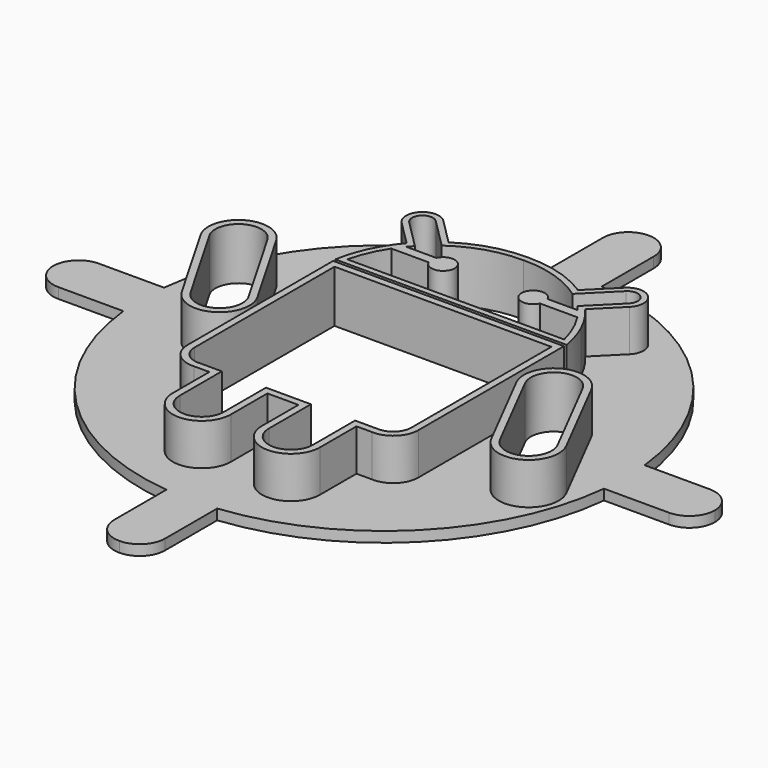
from build123d import *

# Parameters (mm, degrees)
F1_DEPTH = 3
F3_DEPTH = 25
F6_DEPTH = 12
F7_DEPTH = 12
F8_SCALE = 0.5


# Not quite as in the source:
# - a feature of the source that left no trace in its solid (it failed there, or was rolled back) is left out
# - a feature names something its author has since deleted; it is built from what else it names


with BuildPart() as f1:
    # F0 (on Top) → F1 (new body)
    with BuildSketch(Plane.XY):
        with BuildLine():
            ThreePointArc((69.1465082783, -7.3148026297), (69.4358131239, -3.6624855503), (69.532337402, 0))
            ThreePointArc((69.532337402, 0), (69.4358131239, 3.6624855503), (69.1465082783, 7.3148026297))
            ThreePointArc((69.1465082783, 7.3148026297), (49.1667872887, 49.1667872887), (7.3148026297, 69.1465082783))
            ThreePointArc((7.3148026297, 69.1465082783), (0, 69.532337402), (-7.3148026297, 69.1465082783))
            ThreePointArc((-7.3148026297, 69.1465082783), (-49.1667872887, 49.1667872887), (-69.1465082783, 7.3148026297))
            ThreePointArc((-69.1465082783, 7.3148026297), (-69.532337402, 0), (-69.1465082783, -7.3148026297))
            ThreePointArc((-69.1465082783, -7.3148026297), (-49.1667872887, -49.1667872887), (-7.3148026297, -69.1465082783))
            ThreePointArc((-7.3148026297, -69.1465082783), (0, -69.532337402), (7.3148026297, -69.1465082783))
            ThreePointArc((7.3148026297, -69.1465082783), (49.1667872887, -49.1667872887), (69.1465082783, -7.3148026297))
        make_face()
        with BuildLine():
            ThreePointArc((69.1465082783, 7.3148026297), (69.4358131239, 3.6624855503), (69.532337402, 0))
            ThreePointArc((69.532337402, 0), (69.4358131239, -3.6624855503), (69.1465082783, -7.3148026297))
            Line((69.1465082783, -7.3148026297), (87.8831749798, -7.3148026297))
            ThreePointArc((87.8831749798, -7.3148026297), (93.0555215223, -5.1723465425), (95.1979776095, 0))
            ThreePointArc((95.1979776095, 0), (93.0555215223, 5.1723465425), (87.8831749798, 7.3148026297))
            Line((87.8831749798, 7.3148026297), (69.1465082783, 7.3148026297))
        make_face()
        with BuildLine():
            ThreePointArc((-7.3148026297, 69.1465082783), (0, 69.532337402), (7.3148026297, 69.1465082783))
            Line((7.3148026297, 69.1465082783), (7.3148026297, 87.8831749798))
            ThreePointArc((7.3148026297, 87.8831749798), (5.1723465425, 93.0555215223), (0, 95.1979776095))
            ThreePointArc((0, 95.1979776095), (-5.1723465425, 93.0555215223), (-7.3148026297, 87.8831749798))
            Line((-7.3148026297, 87.8831749798), (-7.3148026297, 69.1465082783))
        make_face()
        with BuildLine():
            Line((7.3148026297, -87.8831749798), (7.3148026297, -69.1465082783))
            ThreePointArc((7.3148026297, -69.1465082783), (0, -69.532337402), (-7.3148026297, -69.1465082783))
            Line((-7.3148026297, -69.1465082783), (-7.3148026297, -87.8831749798))
            ThreePointArc((-7.3148026297, -87.8831749798), (-5.1723465425, -93.0555215223), (0, -95.1979776095))
            ThreePointArc((0, -95.1979776095), (5.1723465425, -93.0555215223), (7.3148026297, -87.8831749798))
        make_face()
        with BuildLine():
            ThreePointArc((-69.1465082783, -7.3148026297), (-69.532337402, 0), (-69.1465082783, 7.3148026297))
            Line((-69.1465082783, 7.3148026297), (-87.8831749798, 7.3148026297))
            ThreePointArc((-87.8831749798, 7.3148026297), (-93.0555215223, 5.1723465425), (-95.1979776095, 0))
            ThreePointArc((-95.1979776095, 0), (-93.0555215223, -5.1723465425), (-87.8831749798, -7.3148026297))
            Line((-87.8831749798, -7.3148026297), (-69.1465082783, -7.3148026297))
        make_face()
    extrude(amount=F1_DEPTH)

    # F2 (on face) → F3 (cut)
    with BuildSketch(Plane.XY.offset(3)):
        with BuildLine():
            ThreePointArc((-51.2002213642, 22.0671218808), (-60.2199302878, 24.4839456028), (-62.6367540099, 15.4642366792))
            Line((-62.6367540099, 15.4642366792), (-48.6239641905, -8.8066272438))
            ThreePointArc((-48.6239641905, -8.8066272438), (-39.6042552669, -11.2234509658), (-37.1874315448, -2.2037420422))
            Line((-37.1874315448, -2.2037420422), (-51.2002213642, 22.0671218808))
        make_face()
        with BuildLine():
            Line((0, 21.2101340294), (-31.2078986317, 21.2101340294))
            Line((-31.2078986317, 21.2101340294), (-31.2078986317, -29.1595514864))
            ThreePointArc((-31.2078986317, -29.1595514864), (-29.5536377946, -32.97196325), (-25.6393177885, -34.3680869058))
            Line((-25.6393177885, -34.3680869058), (-19.1715068486, -34.3680869058))
            Line((-19.1715068486, -34.3680869058), (-19.1715068486, -49.4875834141))
            ThreePointArc((-19.1715068486, -49.4875834141), (-12.8196588942, -55.8394313684), (-6.4678109399, -49.4875834141))
            Line((-6.4678109399, -49.4875834141), (-6.4678109399, -34.3680869058))
            Line((-6.4678109399, -34.3680869058), (0, -34.3680869058))
            Line((0, -34.3680869058), (6.4678109399, -34.3680869058))
            Line((6.4678109399, -34.3680869058), (6.4678109399, -49.4875834141))
            ThreePointArc((6.4678109399, -49.4875834141), (12.8196588942, -55.8394313684), (19.1715068486, -49.4875834141))
            Line((19.1715068486, -49.4875834141), (19.1715068486, -34.3680869058))
            Line((19.1715068486, -34.3680869058), (25.6393177885, -34.3680869058))
            ThreePointArc((25.6393177885, -34.3680869058), (29.5536377946, -32.97196325), (31.2078986317, -29.1595514864))
            Line((31.2078986317, -29.1595514864), (31.2078986317, 21.2101340294))
            Line((31.2078986317, 21.2101340294), (0, 21.2101340294))
        make_face()
        with BuildLine():
            ThreePointArc((18.8199247983, 44.2805681259), (9.8819802161, 48.7377457179), (0, 50.1867979765))
            ThreePointArc((0, 50.1867979765), (-9.8819802161, 48.7377457179), (-18.8199247983, 44.2805681259))
            Line((-18.8199247983, 44.2805681259), (-27.3381436975, 52.7987870252))
            ThreePointArc((-27.3381436975, 52.7987870252), (-31.5886529958, 52.7987870252), (-31.5886529958, 48.5482777269))
            Line((-31.5886529958, 48.5482777269), (-23.3639563844, 40.3235811155))
            ThreePointArc((-23.3639563844, 40.3235811155), (-24.0375361692, 39.5906852357), (-24.6877279792, 38.8369633325))
            Line((-24.6877279792, 38.8369633325), (-16.0106173244, 38.8369633325))
            ThreePointArc((-16.0106173244, 38.8369633325), (-9.6142565188, 37.4559091891), (-16.0106173244, 36.0748550456))
            Line((-16.0106173244, 36.0748550456), (-26.7508904588, 36.0748550456))
            ThreePointArc((-26.7508904588, 36.0748550456), (-29.4383336901, 31.1322164007), (-31.2078986317, 25.7917419076))
            Line((-31.2078986317, 25.7917419076), (0, 25.7917419076))
            Line((0, 25.7917419076), (31.2078986317, 25.7917419076))
            ThreePointArc((31.2078986317, 25.7917419076), (29.4383336901, 31.1322164007), (26.7508904588, 36.0748550456))
            Line((26.7508904588, 36.0748550456), (16.0106173244, 36.0748550456))
            ThreePointArc((16.0106173244, 36.0748550456), (9.6142565188, 37.4559091891), (16.0106173244, 38.8369633325))
            Line((16.0106173244, 38.8369633325), (24.6877279792, 38.8369633325))
            ThreePointArc((24.6877279792, 38.8369633325), (24.0375361692, 39.5906852357), (23.3639563844, 40.3235811155))
            Line((23.3639563844, 40.3235811155), (31.5886529958, 48.5482777269))
            ThreePointArc((31.5886529958, 48.5482777269), (31.5886529958, 52.7987870252), (27.3381436975, 52.7987870252))
            Line((27.3381436975, 52.7987870252), (18.8199247983, 44.2805681259))
        make_face()
        with BuildLine():
            ThreePointArc((50.3840297461, -21.2665649388), (59.2676018747, -24.1437740388), (62.1448109747, -15.2602019102))
            Line((62.1448109747, -15.2602019102), (49.3979737771, 9.6987895668))
            ThreePointArc((49.3979737771, 9.6987895668), (40.5144016484, 12.5759986668), (37.6371925484, 3.6924265381))
            Line((37.6371925484, 3.6924265381), (50.3840297461, -21.2665649388))
        make_face()
    extrude(amount=-F3_DEPTH, mode=Mode.SUBTRACT)

    # F4 (on face) → F6 (join)
    with BuildSketch(Plane.XY.offset(3)):
        with BuildLine():
            ThreePointArc((51.1791316906, 10.6084469128), (39.6047443024, 14.3571565803), (35.8560346349, 2.7827691921))
            Line((35.8560346349, 2.7827691921), (48.6028718326, -22.1762222849))
            ThreePointArc((48.6028718326, -22.1762222849), (60.1772592207, -25.9249319523), (63.9259688882, -14.3505445642))
            Line((63.9259688882, -14.3505445642), (51.1791316906, 10.6084469128))
        make_face()
        with BuildLine():
            Line((50.3840297461, -21.2665649388), (37.6371925484, 3.6924265381))
            ThreePointArc((37.6371925484, 3.6924265381), (40.5144016484, 12.5759986668), (49.3979737771, 9.6987895668))
            Line((49.3979737771, 9.6987895668), (62.1448109747, -15.2602019102))
            ThreePointArc((62.1448109747, -15.2602019102), (59.2676018747, -24.1437740388), (50.3840297461, -21.2665649388))
        make_face(mode=Mode.SUBTRACT)
        with BuildLine():
            ThreePointArc((-50.3560149981, -9.8066272438), (-38.6042552669, -12.9555017734), (-35.4553807372, -1.2037420422))
            Line((-35.4553807372, -1.2037420422), (-49.4681705566, 23.0671218808))
            ThreePointArc((-49.4681705566, 23.0671218808), (-61.2199302878, 26.2159964104), (-64.3688048174, 14.4642366792))
            Line((-64.3688048174, 14.4642366792), (-50.3560149981, -9.8066272438))
        make_face()
        with BuildLine():
            Line((-51.2002213642, 22.0671218808), (-37.1874315448, -2.2037420422))
            ThreePointArc((-37.1874315448, -2.2037420422), (-39.6042552669, -11.2234509658), (-48.6239641905, -8.8066272438))
            Line((-48.6239641905, -8.8066272438), (-62.6367540099, 15.4642366792))
            ThreePointArc((-62.6367540099, 15.4642366792), (-60.2199302878, 24.4839456028), (-51.2002213642, 22.0671218808))
        make_face(mode=Mode.SUBTRACT)
    extrude(amount=F6_DEPTH)

    # F4 (on face) → F7 (join)
    with BuildSketch(Plane.XY.offset(3)):
        with BuildLine():
            Line((33.2078986317, -29.1595514864), (33.2078986317, 23.2101340294))
            Line((33.2078986317, 23.2101340294), (-33.2078986317, 23.2101340294))
            Line((-33.2078986317, 23.2101340294), (-33.2078986317, 6.1129540636))
            Line((-33.2078986317, 6.1129540636), (-33.2078986317, -29.1595514864))
            ThreePointArc((-33.2078986317, -29.1595514864), (-30.9461517209, -34.4078767665), (-25.5779123872, -36.3680869058))
            Line((-25.5779123872, -36.3680869058), (-21.1715068486, -36.3680869058))
            Line((-21.1715068486, -36.3680869058), (-21.1715068486, -49.4875834141))
            ThreePointArc((-21.1715068486, -49.4875834141), (-12.8196588942, -57.8394313684), (-4.4678109399, -49.4875834141))
            Line((-4.4678109399, -49.4875834141), (-4.4678109399, -36.3680869058))
            Line((-4.4678109399, -36.3680869058), (4.4678109399, -36.3680869058))
            Line((4.4678109399, -36.3680869058), (4.4678109399, -49.4875834141))
            ThreePointArc((4.4678109399, -49.4875834141), (12.8196588942, -57.8394313684), (21.1715068486, -49.4875834141))
            Line((21.1715068486, -49.4875834141), (21.1715068486, -36.3680869058))
            Line((21.1715068486, -36.3680869058), (25.5779123872, -36.3680869058))
            ThreePointArc((25.5779123872, -36.3680869058), (30.9461517209, -34.4078767665), (33.2078986317, -29.1595514864))
        make_face()
        with BuildLine():
            Line((31.2078986317, 21.2101340294), (31.2078986317, -29.1595514864))
            ThreePointArc((31.2078986317, -29.1595514864), (29.5536377946, -32.97196325), (25.6393177885, -34.3680869058))
            Line((25.6393177885, -34.3680869058), (19.1715068486, -34.3680869058))
            Line((19.1715068486, -34.3680869058), (19.1715068486, -49.4875834141))
            ThreePointArc((19.1715068486, -49.4875834141), (12.8196588942, -55.8394313684), (6.4678109399, -49.4875834141))
            Line((6.4678109399, -49.4875834141), (6.4678109399, -34.3680869058))
            Line((6.4678109399, -34.3680869058), (-6.4678109399, -34.3680869058))
            Line((-6.4678109399, -34.3680869058), (-6.4678109399, -49.4875834141))
            ThreePointArc((-6.4678109399, -49.4875834141), (-12.8196588942, -55.8394313684), (-19.1715068486, -49.4875834141))
            Line((-19.1715068486, -49.4875834141), (-19.1715068486, -34.3680869058))
            Line((-19.1715068486, -34.3680869058), (-25.6393177885, -34.3680869058))
            ThreePointArc((-25.6393177885, -34.3680869058), (-29.5536377946, -32.97196325), (-31.2078986317, -29.1595514864))
            Line((-31.2078986317, -29.1595514864), (-31.2078986317, 21.2101340294))
            Line((-31.2078986317, 21.2101340294), (31.2078986317, 21.2101340294))
        make_face(mode=Mode.SUBTRACT)
        with BuildLine():
            ThreePointArc((-25.707639439, 40.2631011141), (-28.4799020501, 36.5361613442), (-30.7072781513, 32.4600951356))
            ThreePointArc((-30.7072781513, 32.4600951356), (-32.2715668081, 28.3608780057), (-33.284017822, 24.0917419076))
            Line((-33.284017822, 24.0917419076), (33.284017822, 24.0917419076))
            ThreePointArc((33.284017822, 24.0917419076), (32.2715668081, 28.3608780057), (30.7072781513, 32.4600951356))
            ThreePointArc((30.7072781513, 32.4600951356), (28.4799020501, 36.5361613442), (25.707639439, 40.2631011141))
            Line((25.707639439, 40.2631011141), (32.7907345238, 47.3461961989))
            ThreePointArc((32.7907345238, 47.3461961989), (32.7907345238, 54.0008685532), (26.1360621695, 54.0008685532))
            Line((26.1360621695, 54.0008685532), (18.6145214728, 46.4793278565))
            ThreePointArc((18.6145214728, 46.4793278565), (9.708938731, 50.565820618), (0, 51.8869321878))
            ThreePointArc((0, 51.8869321878), (-9.708938731, 50.565820618), (-18.6145214728, 46.4793278565))
            Line((-18.6145214728, 46.4793278565), (-26.1360621695, 54.0008685532))
            ThreePointArc((-26.1360621695, 54.0008685532), (-32.7907345238, 54.0008685532), (-32.7907345238, 47.3461961989))
            Line((-32.7907345238, 47.3461961989), (-25.707639439, 40.2631011141))
        make_face()
        with BuildLine():
            ThreePointArc((16.0106173244, 38.8369633325), (9.6142565188, 37.4559091891), (16.0106173244, 36.0748550456))
            Line((16.0106173244, 36.0748550456), (26.7508904588, 36.0748550456))
            ThreePointArc((26.7508904588, 36.0748550456), (29.4383336901, 31.1322164007), (31.2078986317, 25.7917419076))
            Line((31.2078986317, 25.7917419076), (-31.2078986317, 25.7917419076))
            ThreePointArc((-31.2078986317, 25.7917419076), (-29.4383336901, 31.1322164007), (-26.7508904588, 36.0748550456))
            Line((-26.7508904588, 36.0748550456), (-16.0106173244, 36.0748550456))
            ThreePointArc((-16.0106173244, 36.0748550456), (-9.6142565188, 37.4559091891), (-16.0106173244, 38.8369633325))
            Line((-16.0106173244, 38.8369633325), (-24.6877279792, 38.8369633325))
            ThreePointArc((-24.6877279792, 38.8369633325), (-24.0375361692, 39.5906852357), (-23.3639563844, 40.3235811155))
            Line((-23.3639563844, 40.3235811155), (-31.5886529958, 48.5482777269))
            ThreePointArc((-31.5886529958, 48.5482777269), (-31.5886529958, 52.7987870252), (-27.3381436975, 52.7987870252))
            Line((-27.3381436975, 52.7987870252), (-18.8199247983, 44.2805681259))
            ThreePointArc((-18.8199247983, 44.2805681259), (-9.8819802161, 48.7377457179), (0, 50.1867979765))
            ThreePointArc((0, 50.1867979765), (9.8819802161, 48.7377457179), (18.8199247983, 44.2805681259))
            Line((18.8199247983, 44.2805681259), (27.3381436975, 52.7987870252))
            ThreePointArc((27.3381436975, 52.7987870252), (31.5886529958, 52.7987870252), (31.5886529958, 48.5482777269))
            Line((31.5886529958, 48.5482777269), (23.3639563844, 40.3235811155))
            ThreePointArc((23.3639563844, 40.3235811155), (24.0375361692, 39.5906852357), (24.6877279792, 38.8369633325))
            Line((24.6877279792, 38.8369633325), (16.0106173244, 38.8369633325))
        make_face(mode=Mode.SUBTRACT)
    extrude(amount=F7_DEPTH)


with BuildPart() as f1_1:
    # F8: moved
    add(f1.part.scale(F8_SCALE))


solid = f1_1.part
